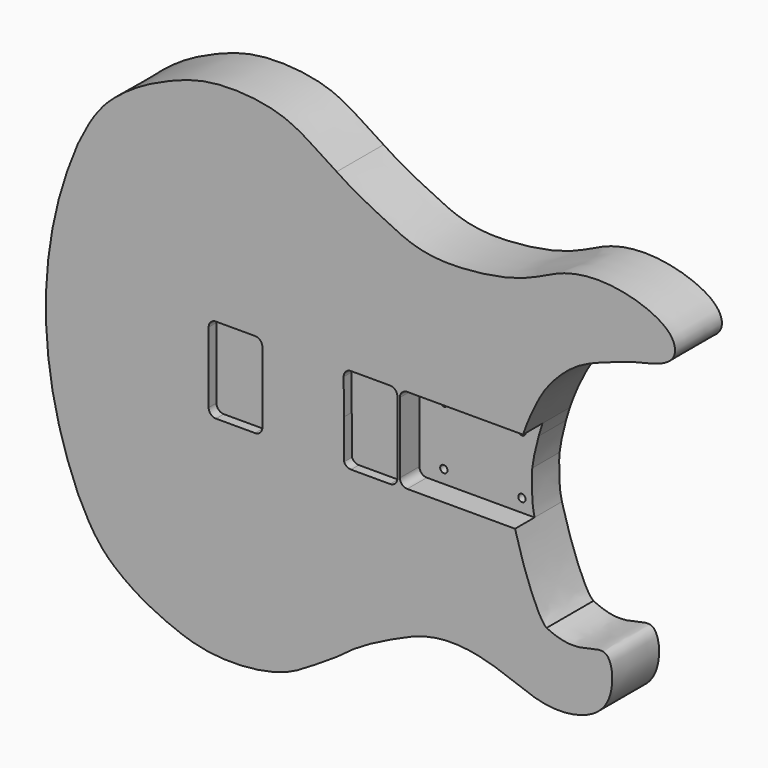
from build123d import *

# Parameters (mm, degrees)
F1_DEPTH = 38.1
F2_DEPTH = 31.75
F0_R     = 2.3876
F0_R_2   = 2.38125
F3_DEPTH = 22.225


# Not quite as in the source:
# - a feature names something its author has since deleted; it is built from what else it names


with BuildPart() as f1:
    # F0 (on Front) → F1 (new body)
    with BuildSketch(Plane.XZ):
        with BuildLine():
            ThreePointArc((-131.7575694882, 99.6186275783), (-147.1851543045, 50.8674279329), (-152.4, 0))
            Line((-152.4, 0), (-46.5183388442, 0))
            Line((-46.5183388442, 0), (-46.5183388442, 22.7864918147))
            ThreePointArc((-46.5183388442, 22.7864918147), (-45.1197151457, 26.1630681162), (-41.7431388442, 27.5616918147))
            Line((-41.7431388442, 27.5616918147), (-16.3431388442, 27.5616918147))
            ThreePointArc((-16.3431388442, 27.5616918147), (-12.9665625427, 26.1630681162), (-11.5679388442, 22.7864918147))
            Line((-11.5679388442, 22.7864918147), (-11.5679388442, 0))
            Line((-11.5679388442, 0), (0, 0))
            Line((0, 0), (41.4718456514, 0))
            Line((41.4718456514, 0), (41.303126597, 22.9711334798))
            ThreePointArc((41.303126597, 22.9711334798), (42.689244329, 26.3703591583), (46.0781977995, 27.7814055627))
            Line((46.0781977995, 27.7814055627), (71.4781977995, 27.7814055627))
            ThreePointArc((71.4781977995, 27.7814055627), (74.854774101, 26.3827818642), (76.2533977995, 23.0062055627))
            Line((76.2533977995, 23.0062055627), (76.2533977995, 0))
            Line((76.2533977995, 0), (77.8774614486, 0))
            Line((77.8774614486, 0), (77.8774614486, 22.987))
            ThreePointArc((77.8774614486, 22.987), (79.2760851471, 26.3635763015), (82.6526614486, 27.7622))
            Line((82.6526614486, 27.7622), (157.8979036882, 27.7622))
            add(Edge.make_bspline(
                [(36.7824863737, 138.8890332392), (44.4611583319, 133.3213390113), (68.3969548865, 121.1035125641), (87.5270580402, 112.0764624619), (112.2586459958, 108.4126359441), (158.3428505383, 114.3006374863), (184.481228653, 131.9333151734), (221.5881831662, 133.8124785147), (257.2301964211, 119.5256611155), (258.0912740588, 98.2783975302), (229.4746316887, 93.2234468873), (220.0898825798, 89.2886493747), (195.8062404605, 81.7121343122), (180.3918257022, 68.5536879314), (169.4275299609, 55.7079954258), (160.8815798819, 36.438372032), (157.8979036882, 27.7622)],
                knots=[0, 0, 0, 0, 0.0831643723, 0.1478611709, 0.2164439231, 0.3102463235, 0.3882453996, 0.4725192478, 0.5552819925, 0.6068068975, 0.6766450792, 0.7244534744, 0.7928300783, 0.8551583748, 0.9161216751, 0.9791881867, 0.9791881867, 0.9791881867, 0.9791881867], degree=3))
            add(Edge.make_bspline(
                [(-131.1600909799, 100.9284788752), (-128.6884574328, 106.0812242447), (-123.1278985731, 116.9514362683), (-113.8799786011, 129.2372204864), (-102.1557652974, 139.0221170642), (-88.619274521, 148.0133254087), (-69.5814006972, 156.9363896764), (-43.4747305791, 165.9507141633), (3.8235065718, 162.7963419752), (21.5299839081, 148.3407105496), (36.7824863737, 138.8890332392)],
                knots=[0.0044092965, 0.0044092965, 0.0044092965, 0.0044092965, 0.1099073913, 0.211197255, 0.3102423882, 0.4130920601, 0.5289321295, 0.6643883739, 0.8333331431, 1, 1, 1, 1], degree=3))
            ThreePointArc((-131.1600909799, 100.9284788752), (-131.4651518463, 100.2764367812), (-131.7575694882, 99.6186275783))
        make_face()
        with BuildLine():
            Line((-46.5183388442, 0), (-152.4, 0))
            ThreePointArc((-152.4, 0), (-147.1112307049, -51.2228813449), (-131.4680695461, -100.2845380932))
            add(Edge.make_bspline(
                [(-131.4680695461, -100.2845380932), (-128.9252759056, -105.6164923147), (-123.2612288852, -116.7743080654), (-113.8799786011, -129.2372204864), (-102.1557652974, -139.0221170642), (-88.619274521, -148.0133254087), (-69.5814006972, -156.9363896764), (-43.4747305791, -165.9507141633), (3.8235065718, -162.7963419752), (21.5299839081, -148.3407105496), (36.7824863737, -138.8890332392)],
                knots=[0, 0, 0, 0, 0.1099073913, 0.211197255, 0.3102423882, 0.4130920601, 0.5289321295, 0.6643883739, 0.8333331431, 1, 1, 1, 1], degree=3))
            add(Edge.make_bspline(
                [(36.7824863737, -138.8890332392), (49.4784885131, -128.6207489175), (70.4922781276, -118.0307589314), (96.0436268745, -106.2354706904), (122.6507034878, -105.6846898276), (150.1677083604, -114.0522068322), (177.1135173345, -126.3284499052), (218.6040772669, -116.6502020858), (216.1429750954, -68.8072129476), (195.7360604991, -86.387796774), (177.0087387061, -79.6971353481), (173.2807112692, -77.9097272706)],
                knots=[0, 0, 0, 0, 0.1217344484, 0.2202709415, 0.3166214553, 0.4177844692, 0.5222537649, 0.6365203065, 0.7384169195, 0.839034432, 0.8633719454, 0.8633719454, 0.8633719454, 0.8633719454], degree=3))
            add(Edge.make_bspline(
                [(173.2807112692, -77.9097272706), (153.0062227083, -68.1890947825), (130.3507500095, -44.145717974), (138.0480290728, -27.8003)],
                knots=[0.8633719454, 0.8633719454, 0.8633719454, 0.8633719454, 0.9957289747, 0.9957289747, 0.9957289747, 0.9957289747], degree=3))
            Line((138.0480290728, -27.8003), (82.6526614486, -27.8003))
            ThreePointArc((82.6526614486, -27.8003), (79.2760851471, -26.4016763015), (77.8774614486, -23.0251))
            Line((77.8774614486, -23.0251), (77.8774614486, 0))
            Line((77.8774614486, 0), (76.2533977995, 0))
            Line((76.2533977995, 0), (76.2533977995, -23.8474573871))
            ThreePointArc((76.2533977995, -23.8474573871), (74.854774101, -27.2240336886), (71.4781977995, -28.6226573871))
            Line((71.4781977995, -28.6226573871), (46.0781977995, -28.6226573871))
            ThreePointArc((46.0781977995, -28.6226573871), (43.4185064384, -27.8133843788), (41.6603129952, -25.6598670802))
            Line((41.6603129952, -25.6598670802), (41.4718456514, 0))
            Line((41.4718456514, 0), (0, 0))
            Line((0, 0), (-11.5679388442, 0))
            Line((-11.5679388442, 0), (-11.5679388442, -23.2383081853))
            ThreePointArc((-11.5679388442, -23.2383081853), (-12.9665625427, -26.6148844869), (-16.3431388442, -28.0135081853))
            Line((-16.3431388442, -28.0135081853), (-41.7431388442, -28.0135081853))
            ThreePointArc((-41.7431388442, -28.0135081853), (-45.1197151457, -26.6148844869), (-46.5183388442, -23.2383081853))
            Line((-46.5183388442, -23.2383081853), (-46.5183388442, 0))
        make_face()
        with BuildLine():
            add(Edge.make_bspline(
                [(173.2807112692, -77.9097272706), (153.0062227083, -68.1890947825), (130.3507500095, -44.145717974), (138.0480290728, -27.8003)],
                knots=[0.8633719454, 0.8633719454, 0.8633719454, 0.8633719454, 0.9957289747, 0.9957289747, 0.9957289747, 0.9957289747], degree=3))
            add(Edge.make_bspline(
                [(173.2807112692, -77.9097272706), (168.1352877555, -74.1051852698), (156.6819668821, -42.6475963813), (156.0319867953, -39.1041042224), (152.7656129543, -27.8003)],
                knots=[0, 0, 0, 0, 0.5604945116, 1, 1, 1, 1], degree=3))
            Line((152.7656129543, -27.8003), (138.0480290728, -27.8003))
        make_face()
    extrude(amount=F1_DEPTH)

    # F0 (on Front) → F3 (join)
    with BuildSketch(Plane.XZ):
        with BuildLine():
            add(Edge.make_bspline(
                [(157.8979036882, 27.7622), (156.9132969547, 24.8990818701), (156.0769836255, 22.1581501372), (155.4495024219, 19.6793314487)],
                knots=[0.9791881867, 0.9791881867, 0.9791881867, 0.9791881867, 1, 1, 1, 1], degree=3))
            Line((157.8979036882, 27.7622), (82.6526614486, 27.7622))
            ThreePointArc((82.6526614486, 27.7622), (79.2760851471, 26.3635763015), (77.8774614486, 22.987))
            Line((77.8774614486, 22.987), (77.8774614486, 0))
            Line((77.8774614486, 0), (151.2687044053, 0))
            add(Edge.make_bspline(
                [(151.2687044053, 0), (151.7371812176, 4.3294030315), (152.8757391691, 10.2827697484), (155.4495024219, 19.6793314487)],
                knots=[0.7265413769, 0.7265413769, 0.7265413769, 0.7265413769, 1, 1, 1, 1], degree=3))
        make_face()
        with Locations((93.7524614486, 18.801197807)):
            Circle(F0_R, mode=Mode.SUBTRACT)
        with Locations((144.5524614486, 18.801197807)):
            Circle(F0_R_2, mode=Mode.SUBTRACT)
        with BuildLine():
            Line((82.6526614486, -27.8003), (138.0480290728, -27.8003))
            Line((138.0480290728, -27.8003), (152.7656129543, -27.8003))
            add(Edge.make_bspline(
                [(152.7656129543, -27.8003), (150.9828500548, -20.8893311334), (151.4595838742, -11.5187694789), (150.7560446319, -4.7377174695), (151.2687044053, 0)],
                knots=[0, 0, 0, 0, 0.427292338, 0.7265413769, 0.7265413769, 0.7265413769, 0.7265413769], degree=3))
            Line((151.2687044053, 0), (77.8774614486, 0))
            Line((77.8774614486, 0), (77.8774614486, -23.0251))
            ThreePointArc((77.8774614486, -23.0251), (79.2760851471, -26.4016763015), (82.6526614486, -27.8003))
        make_face()
        with Locations((93.7524614486, -19.298802193)):
            Circle(F0_R, mode=Mode.SUBTRACT)
        with Locations((144.5524614486, -19.298802193)):
            Circle(F0_R, mode=Mode.SUBTRACT)
    extrude(amount=F3_DEPTH)


with BuildPart() as f2:
    # F0 (on Front) → F2 (new body)
    with BuildSketch(Plane.XZ):
        with BuildLine():
            Line((-46.5183388442, 22.7864918147), (-46.5183388442, 0))
            Line((-46.5183388442, 0), (-11.5679388442, 0))
            Line((-11.5679388442, 0), (-11.5679388442, 22.7864918147))
            ThreePointArc((-11.5679388442, 22.7864918147), (-12.9665625427, 26.1630681162), (-16.3431388442, 27.5616918147))
            Line((-16.3431388442, 27.5616918147), (-41.7431388442, 27.5616918147))
            ThreePointArc((-41.7431388442, 27.5616918147), (-45.1197151457, 26.1630681162), (-46.5183388442, 22.7864918147))
        make_face()
        with BuildLine():
            Line((-11.5679388442, 0), (-46.5183388442, 0))
            Line((-46.5183388442, 0), (-46.5183388442, -23.2383081853))
            ThreePointArc((-46.5183388442, -23.2383081853), (-45.1197151457, -26.6148844869), (-41.7431388442, -28.0135081853))
            Line((-41.7431388442, -28.0135081853), (-16.3431388442, -28.0135081853))
            ThreePointArc((-16.3431388442, -28.0135081853), (-12.9665625427, -26.6148844869), (-11.5679388442, -23.2383081853))
            Line((-11.5679388442, -23.2383081853), (-11.5679388442, 0))
        make_face()
    extrude(amount=F2_DEPTH)


with BuildPart() as f2b:
    # F0 (on Front) → F2, piece 2 (new body)
    with BuildSketch(Plane.XZ):
        with BuildLine():
            Line((41.303126597, 22.9711334798), (41.4718456514, 0))
            Line((41.4718456514, 0), (76.2533977995, 0))
            Line((76.2533977995, 0), (76.2533977995, 23.0062055627))
            ThreePointArc((76.2533977995, 23.0062055627), (74.854774101, 26.3827818642), (71.4781977995, 27.7814055627))
            Line((71.4781977995, 27.7814055627), (46.0781977995, 27.7814055627))
            ThreePointArc((46.0781977995, 27.7814055627), (42.689244329, 26.3703591583), (41.303126597, 22.9711334798))
        make_face()
        with BuildLine():
            Line((76.2533977995, 0), (41.4718456514, 0))
            Line((41.4718456514, 0), (41.6603129952, -25.6598670802))
            ThreePointArc((41.6603129952, -25.6598670802), (43.4185064384, -27.8133843788), (46.0781977995, -28.6226573871))
            Line((46.0781977995, -28.6226573871), (71.4781977995, -28.6226573871))
            ThreePointArc((71.4781977995, -28.6226573871), (74.854774101, -27.2240336886), (76.2533977995, -23.8474573871))
            Line((76.2533977995, -23.8474573871), (76.2533977995, 0))
        make_face()
    extrude(amount=F2_DEPTH)


solid = Compound([f1.part, f2.part, f2b.part])
